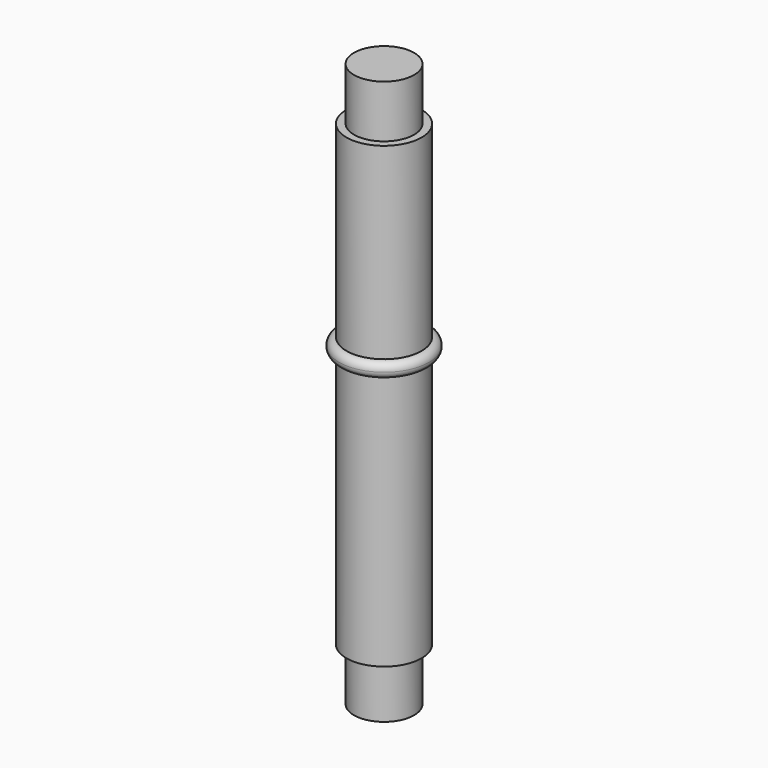
from build123d import *

# Parameters (mm, degrees)
F2_R = 0.99999


# Not quite as in the source:
# - a fillet or chamfer is up to 0.001 mm smaller than in the source, because OpenCascade refuses the exact size


with BuildPart() as f1:
    # F0 (on Front) → F1 (revolve)
    with BuildSketch(Plane.XZ):
        Polygon((4, 75), (0, 75), (0, 0), (4, 0), (4, 7), (5, 7), (5, 41), (6, 41), (6, 43), (5, 43), (5, 68), (4, 68), align=None)
    revolve(axis=Axis((0, 0, 37.5), (0, 0, -1)))

    # F2 (radius 1 in the source; OpenCascade refuses exactly that, so slightly less here)
    f2_edges = [f1.edges().sort_by_distance(p)[0] for p in [
        (-6, 0, 41),
        (-6, 0, 43),
        (6, 0, 42),
    ]]
    fillet(f2_edges, radius=F2_R)


solid = f1.part
